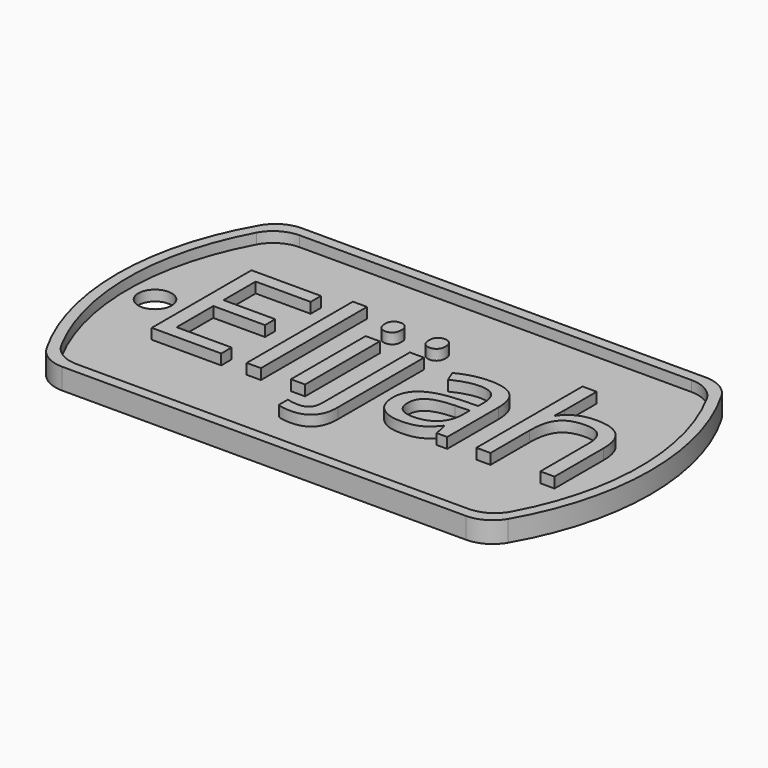
from build123d import *

# Parameters (mm, degrees)
F1_DEPTH     = 1
F3_DEPTH     = 1
F4_R         = 1.5875
F5_DEPTH     = 1
F6_TEXT_SIZE = 16.640705548
F7_DEPTH     = 1


# Not quite as in the source:
# - Text() gives the source's letters only with a copy of the font that has no kerning and outlines rounded to 1/6400 em; it was checked with that copy


with BuildPart() as f1:
    # F0 (on Top) → F1 (new body)
    with BuildSketch(Plane.XY):
        with BuildLine():
            ThreePointArc((-19.2474145991, 14.2875), (-20.8349145991, 13.862130657), (-21.9970452561, 12.7))
            ThreePointArc((-21.9970452561, 12.7), (-25.4, 0), (-21.9970452561, -12.7))
            ThreePointArc((-21.9970452561, -12.7), (-20.8349145991, -13.862130657), (-19.2474145991, -14.2875))
            Line((-19.2474145991, -14.2875), (19.2474145991, -14.2875))
            ThreePointArc((19.2474145991, -14.2875), (20.8349145991, -13.862130657), (21.9970452561, -12.7))
            ThreePointArc((21.9970452561, -12.7), (25.4, 0), (21.9970452561, 12.7))
            ThreePointArc((21.9970452561, 12.7), (20.8349145991, 13.862130657), (19.2474145991, 14.2875))
            Line((19.2474145991, 14.2875), (-19.2474145991, 14.2875))
        make_face()
    extrude(amount=F1_DEPTH)

    # F2 (on face) → F3 (join)
    with BuildSketch(Plane.XY.offset(1)):
        with BuildLine():
            Line((19.2474145991, 14.2875), (-19.2474145991, 14.2875))
            ThreePointArc((-19.2474145991, 14.2875), (-20.8349145991, 13.862130657), (-21.9970452561, 12.7))
            ThreePointArc((-21.9970452561, 12.7), (-25.4, 0), (-21.9970452561, -12.7))
            ThreePointArc((-21.9970452561, -12.7), (-20.8349145991, -13.862130657), (-19.2474145991, -14.2875))
            Line((-19.2474145991, -14.2875), (19.2474145991, -14.2875))
            ThreePointArc((19.2474145991, -14.2875), (20.8349145991, -13.862130657), (21.9970452561, -12.7))
            ThreePointArc((21.9970452561, -12.7), (25.4, 0), (21.9970452561, 12.7))
            ThreePointArc((21.9970452561, 12.7), (20.8349145991, 13.862130657), (19.2474145991, 14.2875))
        make_face()
        with BuildLine():
            ThreePointArc((-21.4526124879, 11.6252061249), (-20.2856017842, 12.8404540819), (-18.6611352482, 13.2875))
            Line((-18.6611352482, 13.2875), (18.6611352482, 13.2875))
            ThreePointArc((18.6611352482, 13.2875), (20.2856017842, 12.8404540819), (21.4526124879, 11.6252061249))
            ThreePointArc((21.4526124879, 11.6252061249), (24.4, 0), (21.4526124879, -11.6252061249))
            ThreePointArc((21.4526124879, -11.6252061249), (20.2856017842, -12.8404540819), (18.6611352482, -13.2875))
            Line((18.6611352482, -13.2875), (-18.6611352482, -13.2875))
            ThreePointArc((-18.6611352482, -13.2875), (-20.2856017842, -12.8404540819), (-21.4526124879, -11.6252061249))
            ThreePointArc((-21.4526124879, -11.6252061249), (-24.4, 0), (-21.4526124879, 11.6252061249))
        make_face(mode=Mode.SUBTRACT)
    extrude(amount=F3_DEPTH)

    # F4 (on face) → F5 (cut)
    with BuildSketch(Plane.XY.offset(1)):
        with Locations((-21.821282804, 0)):
            Circle(F4_R)
    extrude(amount=-F5_DEPTH, mode=Mode.SUBTRACT)

    # F6 (on face) → F7 (join)
    with BuildSketch(Plane.XY.offset(1)):
        with Locations((-19.5825006813, -5.2275997587)):
            Text('Elijah', F6_TEXT_SIZE, font='Open Sans', text_align=(TextAlign.LEFT, TextAlign.BOTTOM))
    extrude(amount=F7_DEPTH)


solid = f1.part
